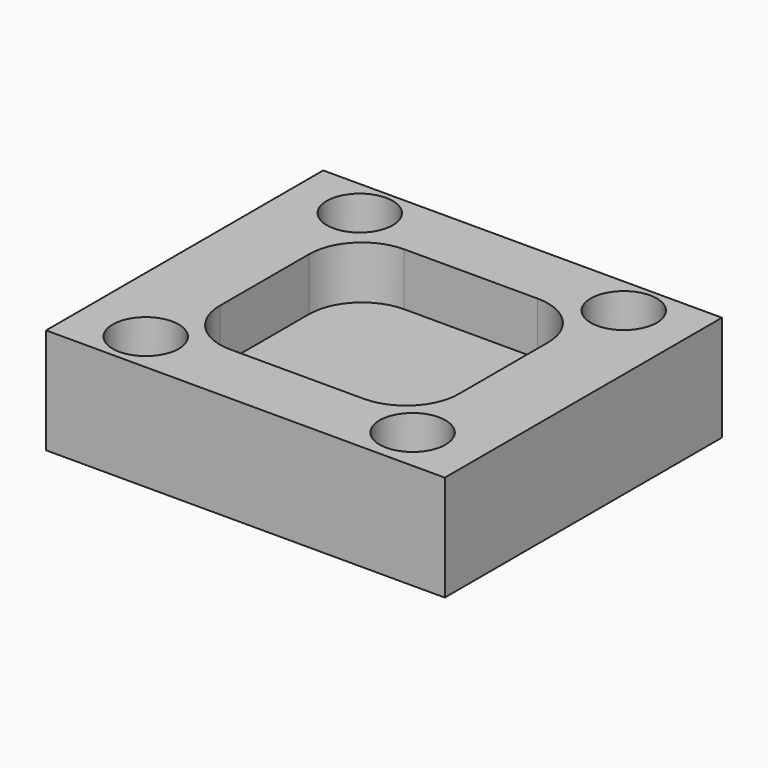
from build123d import *

# Parameters (mm, degrees)
F0_W           = 95.9071815014
F0_H           = 83.329193294
F1_DEPTH       = 25.4
F2_W           = 57.4744343758
F2_H           = 52.2336028516
F3_DEPTH       = 12.7
F4_R           = 12.7
F6_D           = 9.525
F6_CBORE_D     = 15.875
F6_CBORE_DEPTH = 9.525


# Not quite as in the source:
# - a length typed as a fraction of an inch, garbled in the dataset ("3 / 203.2 mm" for 3/8 in), is restored


with BuildPart() as f1:
    # F0 (on Top) → F1 (new body)
    with BuildSketch(Plane.XY):
        Rectangle(F0_W, F0_H)
    extrude(amount=-F1_DEPTH)

    # F2 (on face) → F3 (cut)
    with BuildSketch(Plane.XY):
        Rectangle(F2_W, F2_H)
    extrude(amount=-F3_DEPTH, mode=Mode.SUBTRACT)

    # F4
    f4_edges = [f1.edges().sort_by_distance(p)[0] for p in [
        (-28.737217, 26.116801, -6.35),
        (28.737217, 26.116801, -6.35),
        (-28.737217, -26.116801, -6.35),
        (28.737217, -26.116801, -6.35),
    ]]
    fillet(f4_edges, radius=F4_R)

    # F6 (through all)
    with Locations(Plane.XY):
        with Locations((-31.75, 32.4055403471), (31.75, 32.4055403471), (31.75, -31.0944596529), (-31.75, -31.9523103535)):
            CounterBoreHole(F6_D / 2, F6_CBORE_D / 2, F6_CBORE_DEPTH)


solid = f1.part
